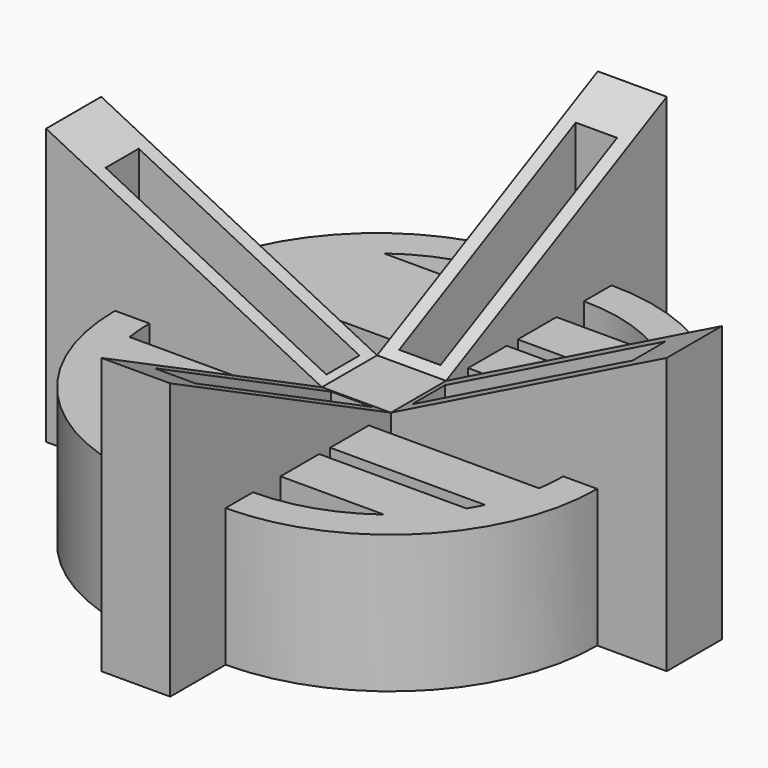
from build123d import *

# Parameters (mm, degrees)
F0_W      = 12.7
F0_H      = 12.7
F1_DEPTH  = 50.8
F3_DEPTH  = 25.4
F5_DEPTH  = 25.4
F7_DEPTH  = 12.7
F9_DEPTH  = 25.4
F12_DEPTH = 25.4
F13_W     = 40.64
F13_H     = 7.62
F15_W     = 7.62
F15_H     = 40.64
F11_W     = 7.62
F11_H     = 40.64
F14_W     = 40.64
F14_H     = 7.62
F16_DEPTH = 43.18


# Not quite as in the source:
# - a feature names something its author has since deleted; it is built from what else it names


with BuildPart() as f1:
    # F0 (on Top) → F1 (new body)
    with BuildSketch(Plane.XY):
        Polygon((0, 12.7), (0, 0), (31.75, 0), (38.0062268819, 0), (50.8, 0), (50.8, 12.7), (38.1, 12.7), (31.75, 12.7), align=None)
        Polygon((0, -5.08), (0, 0), (-12.7, 0), (-12.7, -5.08), (-12.7, -13.97), (-12.7, -16.51), (-12.7, -25.4), (-12.7, -31.75), (-12.7, -38.1), (-12.7, -50.8), (0, -50.8), (0, -38.0530845557), (0, -31.75), (0, -25.4), (0, -16.51), (0, -13.97), align=None)
        Polygon((-12.7, 12.7), (0, 12.7), (0, 17.78), (0, 26.67), (0, 29.21), (0, 38.1), (0, 44.45), (0, 50.8), (0, 63.5), (-12.7, 63.5), (-12.7, 50.8), (-12.7, 44.45), (-12.7, 38.1), (-12.7, 26.67), (-12.7, 17.78), align=None)
        Polygon((-44.45, 0), (-12.7, 0), (-12.7, 12.7), (-44.45, 12.7), (-50.8, 12.7), (-63.5, 12.7), (-63.5, 0), (-50.8, 0), align=None)
        with Locations((-6.35, 6.35)):
            Rectangle(F0_W, F0_H)
    extrude(amount=F1_DEPTH)

    # F2 (on face) → F3 (cut)
    with BuildSketch(Plane.XZ):
        Polygon((-63.5, 50.8), (-12.7, 25.4), (-12.7, 50.8), align=None)
    extrude(amount=-F3_DEPTH, mode=Mode.SUBTRACT)

    # F4 (on face) → F5 (cut)
    with BuildSketch(Plane(origin=(-12.7, 0, 0), x_dir=(0, -1, 0), z_dir=(-1, 0, 0))):
        Polygon((0, 50.8), (0, 25.4), (50.8, 50.8), align=None)
    extrude(amount=-F5_DEPTH, mode=Mode.SUBTRACT)

    # F6 (on face) → F7 (cut)
    with BuildSketch(Plane(origin=(-12.7, 0, 0), x_dir=(0, -1, 0), z_dir=(-1, 0, 0))):
        Polygon((-12.7, 25.4), (0, 25.4), (0, 50.8), (-63.5, 50.8), align=None)
    extrude(amount=-F7_DEPTH, mode=Mode.SUBTRACT)

    # F8 (on face) → F9 (cut)
    with BuildSketch(Plane(origin=(0, 12.7, 0), x_dir=(-1, 0, 0), z_dir=(0, 1, 0))):
        Polygon((-50.8, 50.8), (0, 25.4), (0, 50.8), align=None)
    extrude(amount=-F9_DEPTH, mode=Mode.SUBTRACT)

    # F0 (on Top) → F12 (join)
    with BuildSketch(Plane.XY):
        with BuildLine():
            Line((38.0062268819, 0), (31.75, 0))
            ThreePointArc((31.75, 0), (31.6475760941, -2.5482204312), (31.3409652053, -5.08))
            ThreePointArc((31.3409652053, -5.08), (30.2545088643, -9.6294960085), (28.5114292872, -13.97))
            ThreePointArc((28.5114292872, -13.97), (27.8445816489, -15.2558766643), (27.1197787602, -16.51))
            ThreePointArc((27.1197787602, -16.51), (23.5089375066, -21.339924023), (19.05, -25.4))
            ThreePointArc((19.05, -25.4), (10.040231571, -30.1206947131), (0, -31.75))
            Line((0, -31.75), (0, -38.0530845557))
            ThreePointArc((0, -38.0530845557), (26.8772997991, -26.8910325481), (38.0062268819, 0))
        make_face()
        with BuildLine():
            ThreePointArc((31.3409652053, 17.78), (31.6475760941, 15.2482204312), (31.75, 12.7))
            Line((31.75, 12.7), (38.1, 12.7))
            ThreePointArc((38.1, 12.7), (26.9407683632, 39.6407683632), (0, 50.8))
            Line((0, 50.8), (0, 44.45))
            ThreePointArc((0, 44.45), (10.040231571, 42.8206947131), (19.05, 38.1))
            ThreePointArc((19.05, 38.1), (23.5089375066, 34.039924023), (27.1197787602, 29.21))
            ThreePointArc((27.1197787602, 29.21), (27.8445816489, 27.9558766643), (28.5114292872, 26.67))
            ThreePointArc((28.5114292872, 26.67), (30.2545088643, 22.3294960085), (31.3409652053, 17.78))
        make_face()
        with BuildLine():
            Line((-12.7, -13.97), (-12.7, -5.08))
            Line((-12.7, -5.08), (-44.0409652053, -5.08))
            ThreePointArc((-44.0409652053, -5.08), (-44.3475760941, -2.5482204312), (-44.45, 0))
            Line((-44.45, 0), (-50.8, 0))
            ThreePointArc((-50.8, 0), (-39.6407683632, -26.9407683632), (-12.7, -38.1))
            Line((-12.7, -38.1), (-12.7, -31.75))
            ThreePointArc((-12.7, -31.75), (-22.740231571, -30.1206947131), (-31.75, -25.4))
            ThreePointArc((-31.75, -25.4), (-36.2089375066, -21.339924023), (-39.8197787602, -16.51))
            ThreePointArc((-39.8197787602, -16.51), (-40.5445816489, -15.2558766643), (-41.2114292872, -13.97))
            Line((-41.2114292872, -13.97), (-12.7, -13.97))
        make_face()
        with BuildLine():
            Line((-50.8, 12.7), (-44.45, 12.7))
            ThreePointArc((-44.45, 12.7), (-44.3475760941, 15.2482204312), (-44.0409652053, 17.78))
            ThreePointArc((-44.0409652053, 17.78), (-42.9545088643, 22.3294960085), (-41.2114292872, 26.67))
            ThreePointArc((-41.2114292872, 26.67), (-37.1577924997, 32.9454658143), (-31.75, 38.1))
            ThreePointArc((-31.75, 38.1), (-22.740231571, 42.8206947131), (-12.7, 44.45))
            Line((-12.7, 44.45), (-12.7, 50.8))
            ThreePointArc((-12.7, 50.8), (-39.6407683632, 39.6407683632), (-50.8, 12.7))
        make_face()
        with BuildLine():
            Line((-12.7, -25.4), (-12.7, -16.51))
            Line((-12.7, -16.51), (-39.8197787602, -16.51))
            ThreePointArc((-39.8197787602, -16.51), (-36.2089375066, -21.339924023), (-31.75, -25.4))
            Line((-31.75, -25.4), (-12.7, -25.4))
        make_face()
        with BuildLine():
            Line((0, 38.1), (0, 29.21))
            Line((0, 29.21), (27.1197787602, 29.21))
            ThreePointArc((27.1197787602, 29.21), (23.5089375066, 34.039924023), (19.05, 38.1))
            Line((19.05, 38.1), (0, 38.1))
        make_face()
        with BuildLine():
            Line((0, 26.67), (0, 17.78))
            Line((0, 17.78), (31.3409652053, 17.78))
            ThreePointArc((31.3409652053, 17.78), (30.2545088643, 22.3294960085), (28.5114292872, 26.67))
            Line((28.5114292872, 26.67), (0, 26.67))
        make_face()
        with BuildLine():
            Line((-41.2114292872, 26.67), (-12.7, 26.67))
            Line((-12.7, 26.67), (-12.7, 38.1))
            Line((-12.7, 38.1), (-31.75, 38.1))
            ThreePointArc((-31.75, 38.1), (-37.1577924997, 32.9454658143), (-41.2114292872, 26.67))
        make_face()
        with BuildLine():
            Line((-44.0409652053, 17.78), (-12.7, 17.78))
            Line((-12.7, 17.78), (-12.7, 26.67))
            Line((-12.7, 26.67), (-41.2114292872, 26.67))
            ThreePointArc((-41.2114292872, 26.67), (-42.9545088643, 22.3294960085), (-44.0409652053, 17.78))
        make_face()
        with BuildLine():
            Line((31.3409652053, -5.08), (0, -5.08))
            Line((0, -5.08), (0, -13.97))
            Line((0, -13.97), (28.5114292872, -13.97))
            ThreePointArc((28.5114292872, -13.97), (30.2545088643, -9.6294960085), (31.3409652053, -5.08))
        make_face()
        with BuildLine():
            Line((27.1197787602, -16.51), (0, -16.51))
            Line((0, -16.51), (0, -25.4))
            Line((0, -25.4), (19.05, -25.4))
            ThreePointArc((19.05, -25.4), (23.5089375066, -21.339924023), (27.1197787602, -16.51))
        make_face()
    extrude(amount=F12_DEPTH)

    # F13 (on offset) + F15 (on offset) + F11 (on offset) + F14 (on offset) → F16 (cut)
    with BuildSketch(Plane.XY.offset(52.324)):
        with Locations((22.1610166958, 6.35)):
            Rectangle(F13_W, F13_H)
    with BuildSketch(Plane.XY.offset(52.324)):
        with Locations((-6.35, -21.4313176799)):
            Rectangle(F15_W, F15_H)
    with BuildSketch(Plane.XY.offset(52.324)):
        with Locations((-6.35, 34.922975541)):
            Rectangle(F11_W, F11_H)
    with BuildSketch(Plane.XY.offset(52.324)):
        with Locations((-34.2408475804, 6.35)):
            Rectangle(F14_W, F14_H)
    extrude(amount=-F16_DEPTH, mode=Mode.SUBTRACT)


solid = f1.part
